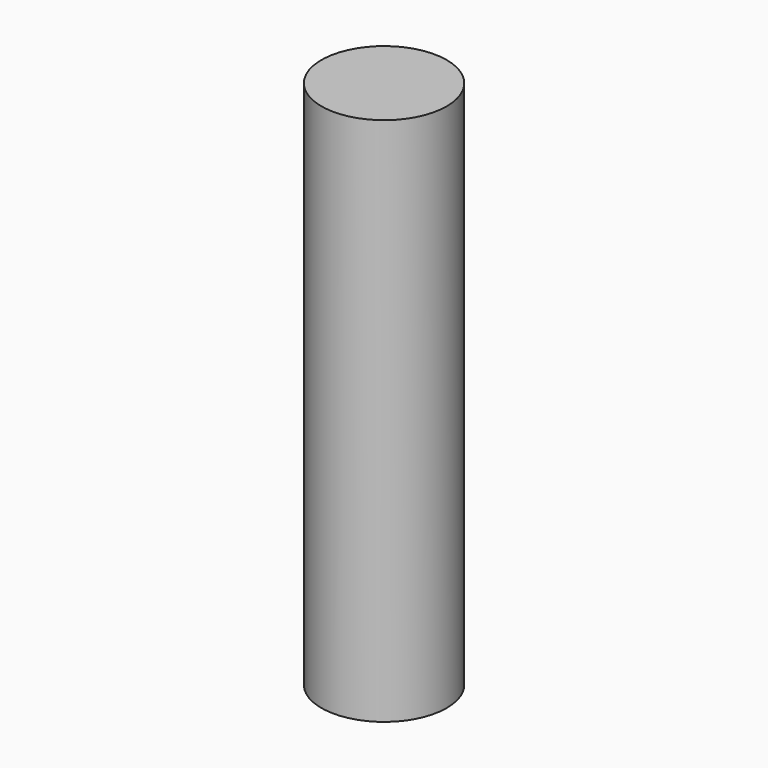
from build123d import *

# Parameters (mm, degrees)
F0_R     = 11.2395
F1_DEPTH = 94.996


# Not quite as in the source:
# - the program builds the solid bodies; features that only make, move or delete a surface that nothing else refers to are left out


with BuildPart() as f1:
    # F0 (on Top) → F1 (new body)
    with BuildSketch(Plane.XY):
        Circle(F0_R)
    extrude(amount=F1_DEPTH)


solid = f1.part
